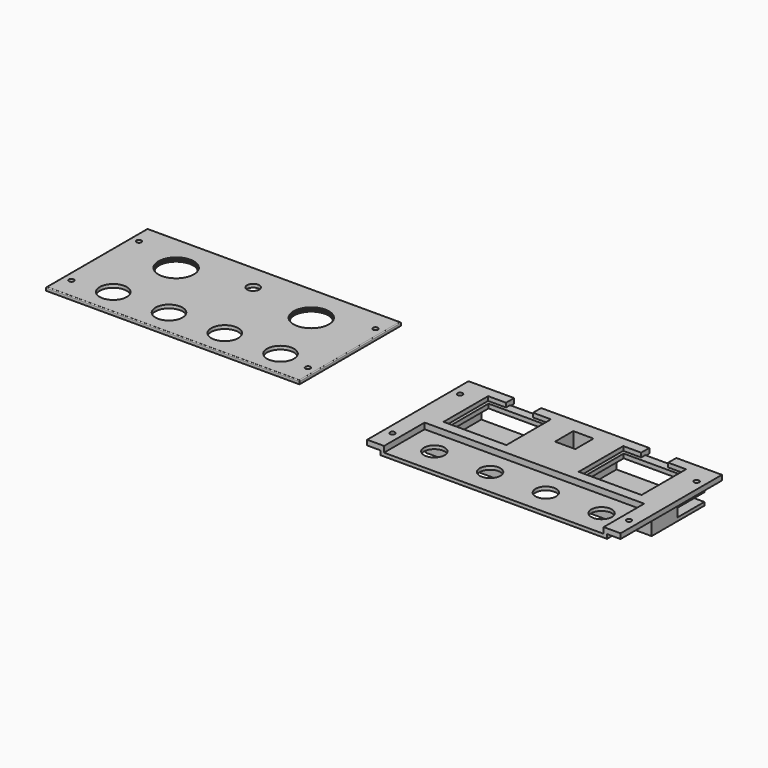
from build123d import *

# Parameters (mm, degrees)
F0_W      = 150
F0_H      = 75
F0_R      = 1.5
F0_R_2    = 6.1
F0_W_2    = 33.5
F0_H_2    = 29
F0_W_3    = 12
F0_H_3    = 8
F1_DEPTH  = 2
F2_W      = 10
F2_H      = 75
F3_DEPTH  = 3.5
F4_W      = 8
F4_H      = 2.5
F5_DEPTH  = 80
F6_W      = 130
F6_H      = 45
F6_W_2    = 33.5
F6_H_2    = 29
F6_W_3    = 12
F6_H_3    = 13.5
F7_DEPTH  = 3.5
F8_W      = 33.5
F8_H      = 29
F8_W_2    = 16
F8_H_2    = 9
F8_H_3    = 6
F9_DEPTH  = 2.5
F10_W     = 150
F10_H     = 75
F10_R     = 1.5
F10_R_2   = 8
F10_R_3   = 10
F10_R_4   = 3.6
F11_DEPTH = 2
F12_R     = 10.5
F13_DEPTH = 1
F14_W     = 26
F14_H     = 25
F15_DEPTH = 4.5
F16_W     = 12
F16_H     = 13.5
F17_DEPTH = 9
F18_W     = 134
F18_H     = 3
F19_DEPTH = 2.5
F20_W     = 54
F20_H     = 39
F20_W_2   = 33.5
F20_H_2   = 29
F21_DEPTH = 12
F22_W     = 50
F22_H     = 10.5
F23_DEPTH = 37
F24_R     = 1.5
F25_DEPTH = 25
F26_W     = 16
F26_H     = 3
F27_DEPTH = 3
F28_R     = 0.5
F30_W     = 20
F30_H     = 5
F29_W     = 20
F29_H     = 5
F31_DEPTH = 4
F32_W     = 2
F32_H     = 20
F33_DEPTH = 0.5


# Not quite as in the source:
# - a feature names something its author has since deleted; it is built from what else it names


with BuildPart() as f1:
    # F0 (on Top) → F1 (new body)
    with BuildSketch(Plane.XY):
        Rectangle(F0_W, F0_H)
        with Locations((-70, -25)):
            Circle(F0_R, mode=Mode.SUBTRACT)
        with Locations((-47.6297214627, -22)):
            Circle(F0_R_2, mode=Mode.SUBTRACT)
        with Locations((-14.6297214627, -22)):
            Circle(F0_R_2, mode=Mode.SUBTRACT)
        with Locations((18.3702785373, -22)):
            Circle(F0_R_2, mode=Mode.SUBTRACT)
        with Locations((51.3702785373, -22)):
            Circle(F0_R_2, mode=Mode.SUBTRACT)
        with Locations((70, -25)):
            Circle(F0_R, mode=Mode.SUBTRACT)
        with Locations((-40, 15)):
            Rectangle(F0_W_2, F0_H_2, mode=Mode.SUBTRACT)
        with Locations((-70, 25)):
            Circle(F0_R, mode=Mode.SUBTRACT)
        with Locations((40, 15)):
            Rectangle(F0_W_2, F0_H_2, mode=Mode.SUBTRACT)
        Polygon((6, 18), (6, 15.25), (-6, 15.25), (-6, 18), (-6, 26), (-6, 28.75), (6, 28.75), (6, 26), align=None, mode=Mode.SUBTRACT)
        with Locations((70, 25)):
            Circle(F0_R, mode=Mode.SUBTRACT)
        with Locations((0, 22)):
            Rectangle(F0_W_3, F0_H_3)
    extrude(amount=F1_DEPTH)

    # F2 (on face) → F3 (join)
    with BuildSketch(Plane.XY.offset(2)):
        with Locations((-70, 0)):
            Rectangle(F2_W, F2_H)
        with Locations((70, 0)):
            Rectangle(F2_W, F2_H)
    extrude(amount=F3_DEPTH)

    # F4 (on face) → F5 (cut)
    with BuildSketch(Plane.XZ.offset(37.5)):
        with Locations((-71, 1.25)):
            Rectangle(F4_W, F4_H)
        with Locations((71, 1.25)):
            Rectangle(F4_W, F4_H)
    extrude(amount=-F5_DEPTH, mode=Mode.SUBTRACT)

    # F6 (on face) → F7 (join)
    with BuildSketch(Plane.XY.offset(2)):
        with Locations((0, 15)):
            Rectangle(F6_W, F6_H)
        with Locations((-40, 15)):
            Rectangle(F6_W_2, F6_H_2, mode=Mode.SUBTRACT)
        with Locations((0, 22)):
            Rectangle(F6_W_3, F6_H_3, mode=Mode.SUBTRACT)
        with Locations((40, 15)):
            Rectangle(F6_W_2, F6_H_2, mode=Mode.SUBTRACT)
    extrude(amount=F7_DEPTH)

    # F8 (on face) → F9 (cut)
    with BuildSketch(Plane.XY.offset(5.5)):
        Polygon((-58.6, -1.5), (-21.4, -1.5), (-21.4, 31.5), (-32, 31.5), (-48, 31.5), (-58.6, 31.5), align=None)
        with Locations((-40, 15)):
            Rectangle(F8_W, F8_H, mode=Mode.SUBTRACT)
        Polygon((48, 31.5), (32, 31.5), (21.4, 31.5), (21.4, -1.5), (58.6, -1.5), (58.6, 31.5), align=None)
        with Locations((40, 15)):
            Rectangle(F8_W, F8_H, mode=Mode.SUBTRACT)
        with Locations((-40, 42)):
            Rectangle(F8_W_2, F8_H_2)
        with Locations((40, 42)):
            Rectangle(F8_W_2, F8_H_2)
        with Locations((-40, 34.5)):
            Rectangle(F8_W_2, F8_H_3)
        with Locations((40, 34.5)):
            Rectangle(F8_W_2, F8_H_3)
    extrude(amount=-F9_DEPTH, mode=Mode.SUBTRACT)

    # F14 (on face) + F0 (on Top) → F15 (join)
    with BuildSketch(Plane.XY):
        with Locations((0, 22)):
            Rectangle(F14_W, F14_H)
        Polygon((6, 28.75), (6, 26), (6, 18), (6, 15.25), (-6, 15.25), (-6, 18), (-6, 26), (-6, 28.75), align=None, mode=Mode.SUBTRACT)
    with BuildSketch(Plane.XY):
        with Locations((0, 22)):
            Rectangle(F0_W_3, F0_H_3)
    extrude(amount=-F15_DEPTH)

    # F16 (on face) → F17 (cut)
    with BuildSketch(Plane.XY.offset(5.5)):
        with Locations((0, 22)):
            Rectangle(F16_W, F16_H)
    extrude(amount=-F17_DEPTH, mode=Mode.SUBTRACT)

    # F18 (on face) → F19 (cut)
    with BuildSketch(Plane.XY):
        with Locations((0, 36)):
            Rectangle(F18_W, F18_H)
    extrude(amount=F19_DEPTH, mode=Mode.SUBTRACT)

    # F20 (on face) → F21 (join)
    with BuildSketch(Plane.XY):
        with Locations((40, 15)):
            Rectangle(F20_W, F20_H)
        with Locations((40, 15)):
            Rectangle(F20_W_2, F20_H_2, mode=Mode.SUBTRACT)
        with Locations((-40, 15)):
            Rectangle(F20_W, F20_H)
        with Locations((-40, 15)):
            Rectangle(F20_W_2, F20_H_2, mode=Mode.SUBTRACT)
        with Locations((40, 15)):
            Rectangle(F20_W_2, F20_H_2)
        with Locations((-40, 15)):
            Rectangle(F20_W_2, F20_H_2)
    extrude(amount=-F21_DEPTH)

    # F22 (on face) → F23 (cut)
    with BuildSketch(Plane(origin=(0, 34.5, 0), x_dir=(-1, 0, 0), z_dir=(0, 1, 0))):
        with Locations((-40, -4.75)):
            Rectangle(F22_W, F22_H)
        with Locations((40, -4.75)):
            Rectangle(F22_W, F22_H)
    extrude(amount=-F23_DEPTH, mode=Mode.SUBTRACT)

    # F24 (on face) → F25 (cut)
    with BuildSketch(Plane.XY.offset(5.5)):
        with Locations((-70, 25)):
            Circle(F24_R)
        with Locations((-70, -25)):
            Circle(F24_R)
        with Locations((70, 25)):
            Circle(F24_R)
        with Locations((70, -25)):
            Circle(F24_R)
    extrude(amount=-F25_DEPTH, mode=Mode.SUBTRACT)

    # F26 (on face) → F27 (cut)
    with BuildSketch(Plane.XY.offset(3)):
        with Locations((-40, 36)):
            Rectangle(F26_W, F26_H)
        with Locations((40, 36)):
            Rectangle(F26_W, F26_H)
    extrude(amount=-F27_DEPTH, mode=Mode.SUBTRACT)

    # F30 (on face) + F29 (on face) → F31 (cut)
    with BuildSketch(Plane.YZ.offset(67)):
        with Locations((24.5, -7.5)):
            Rectangle(F30_W, F30_H)
    with BuildSketch(Plane.YZ.offset(-13)):
        with Locations((24.5, -7.5)):
            Rectangle(F29_W, F29_H)
    extrude(amount=-F31_DEPTH, mode=Mode.SUBTRACT)

    # F32 (on face) → F33 (cut)
    with BuildSketch(Plane(origin=(0, 0, -5), x_dir=(1, 0, 0), z_dir=(0, 0, -1))):
        with Locations((-14, -24.5)):
            Rectangle(F32_W, F32_H)
    extrude(amount=-F33_DEPTH, mode=Mode.SUBTRACT)


with BuildPart() as f11:
    # F10 (on Top) → F11 (new body)
    with BuildSketch(Plane.XY):
        with Locations((-215.6192851201, 31.9309936473)):
            Rectangle(F10_W, F10_H)
        with Locations((-285.6192851201, 6.9309936473)):
            Circle(F10_R, mode=Mode.SUBTRACT)
        with Locations((-263.2490065828, 9.9309936473)):
            Circle(F10_R_2, mode=Mode.SUBTRACT)
        with Locations((-230.2490065828, 9.9309936473)):
            Circle(F10_R_2, mode=Mode.SUBTRACT)
        with Locations((-197.2490065828, 9.9309936473)):
            Circle(F10_R_2, mode=Mode.SUBTRACT)
        with Locations((-164.2490065828, 9.9309936473)):
            Circle(F10_R_2, mode=Mode.SUBTRACT)
        with Locations((-145.6192851201, 6.9309936473)):
            Circle(F10_R, mode=Mode.SUBTRACT)
        with Locations((-255.6192851201, 46.9309936473)):
            Circle(F10_R_3, mode=Mode.SUBTRACT)
        with Locations((-285.6192851201, 56.9309936473)):
            Circle(F10_R, mode=Mode.SUBTRACT)
        with Locations((-175.6192851201, 46.9309936473)):
            Circle(F10_R_3, mode=Mode.SUBTRACT)
        with Locations((-215.6192851201, 53.9309936473)):
            Circle(F10_R_4, mode=Mode.SUBTRACT)
        with Locations((-145.6192851201, 56.9309936473)):
            Circle(F10_R, mode=Mode.SUBTRACT)
    extrude(amount=F11_DEPTH)

    # F12 (on face) → F13 (cut)
    with BuildSketch(Plane.XY.offset(2)):
        with Locations((-255.6192851201, 46.9309936473)):
            Circle(F12_R)
        with Locations((-175.6192851201, 46.9309936473)):
            Circle(F12_R)
    extrude(amount=-F13_DEPTH, mode=Mode.SUBTRACT)

    # F28
    f28_edges = [f11.edges().sort_by_distance(p)[0] for p in [
        (-290.619285, 31.930994, 2),
        (-215.619285, 69.430994, 2),
        (-140.619285, 31.930994, 2),
        (-215.619285, -5.569006, 2),
    ]]
    fillet(f28_edges, radius=F28_R)


solid = Compound([f1.part, f11.part])
